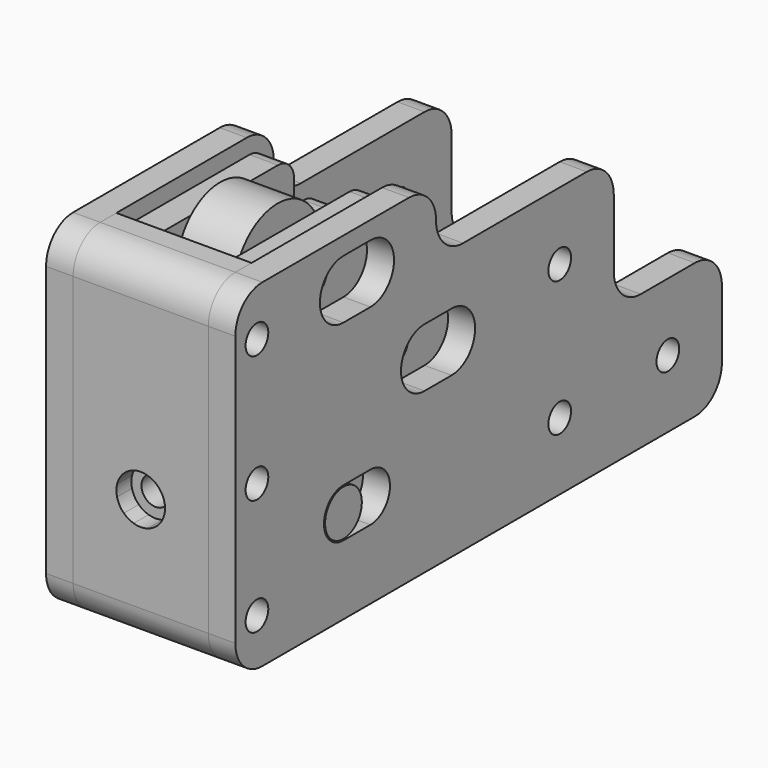
from build123d import *

# Parameters (mm, degrees)
F1_START      = 10
F0_R          = 2.1
F1_DEPTH      = 4
F2_START      = -10
F2_DEPTH      = 4
F3_R          = 8
F3_R_2        = 2.5
F4_DEPTH      = 4.25
F4_DEPTH_BACK = 4.25
F5_DEPTH      = 10
F5_DEPTH_BACK = 10
F6_W          = 3
F6_H          = 39.1219552991
F7_DEPTH      = 9.5
F7_DEPTH_BACK = 9.5
F8_START      = 5.3
F6_R          = 3.4
F6_R_2        = 4.25
F6_R_3        = 2.6
F8_DEPTH      = 4.2
F9_START      = -5.3
F9_DEPTH      = 4.2
F10_START     = 9.5
F10_DEPTH     = 4.5
F11_START     = -9.5
F11_DEPTH     = 4.5
F12_START     = 4.5
F12_DEPTH     = 0.8
F13_START     = -4.5
F13_DEPTH     = 0.8
F14_SIZE      = 0.79999
F15_R         = 2.1
F16_DEPTH     = 56.7675373241
F17_DEPTH     = 47
F18_START     = 54
F18_DEPTH     = 2.7675373241


# Not quite as in the source:
# - a fillet or chamfer is up to 0.001 mm smaller than in the source, because OpenCascade refuses the exact size
# - a feature names something its author has since deleted; it is built from what else it names


with BuildPart() as f1:
    # F0 (on Right) → F1 (new body)
    with BuildSketch(Plane.YZ.offset(F1_START)):
        with BuildLine():
            ThreePointArc((-56.7665373241, -19.1860739807), (-55.30207123, -22.7216078866), (-51.7665373241, -24.1860739807))
            Line((-51.7665373241, -24.1860739807), (-48.7665373241, -24.1860739807))
            Line((-48.7665373241, -24.1860739807), (-48.7665373241, 25.8139260193))
            Line((-48.7665373241, 25.8139260193), (-51.7665373241, 25.8139260193))
            ThreePointArc((-51.7665373241, 25.8139260193), (-55.30207123, 24.3494599252), (-56.7665373241, 20.8139260193))
            Line((-56.7665373241, 20.8139260193), (-56.7665373241, -19.1860739807))
        make_face()
        with Locations((-52.7665373241, -17.1860739807)):
            Circle(F0_R, mode=Mode.SUBTRACT)
        with Locations((-52.7665373241, 0)):
            Circle(F0_R, mode=Mode.SUBTRACT)
        with Locations((-52.7665373241, 18.8139260193)):
            Circle(F0_R, mode=Mode.SUBTRACT)
        with BuildLine():
            Line((-48.7665373241, 25.8139260193), (-48.7665373241, -24.1860739807))
            Line((-48.7665373241, -24.1860739807), (28.2334626759, -24.1860739807))
            ThreePointArc((28.2334626759, -24.1860739807), (31.7689965819, -22.7216078866), (33.2334626759, -19.1860739807))
            Line((33.2334626759, -19.1860739807), (33.2334626759, -9.1860739807))
            ThreePointArc((33.2334626759, -9.1860739807), (31.7689965819, -5.6505400748), (28.2334626759, -4.1860739807))
            Line((28.2334626759, -4.1860739807), (18.2334626759, -4.1860739807))
            ThreePointArc((18.2334626759, -4.1860739807), (14.69792877, -2.7216078866), (13.2334626759, 0.8139260193))
            Line((13.2334626759, 0.8139260193), (13.2334626759, 10.8139260193))
            ThreePointArc((13.2334626759, 10.8139260193), (11.7689965819, 14.3494599252), (8.2334626759, 15.8139260193))
            Line((8.2334626759, 15.8139260193), (-14.6415373241, 15.8139260193))
            ThreePointArc((-14.6415373241, 15.8139260193), (-18.17707123, 17.2783921134), (-19.6415373241, 20.8139260193))
            ThreePointArc((-19.6415373241, 20.8139260193), (-21.1060034181, 24.3494599252), (-24.6415373241, 25.8139260193))
            Line((-24.6415373241, 25.8139260193), (-48.7665373241, 25.8139260193))
        make_face()
        with BuildLine():
            ThreePointArc((-36.7665373241, -13.9080292798), (-40.3665373241, -10.3080292798), (-36.7665373241, -6.7080292798))
            Line((-36.7665373241, -6.7080292798), (-31.7665373241, -6.7080292798))
            ThreePointArc((-31.7665373241, -6.7080292798), (-28.1665373241, -10.3080292798), (-31.7665373241, -13.9080292798))
            Line((-31.7665373241, -13.9080292798), (-36.7665373241, -13.9080292798))
        make_face(mode=Mode.SUBTRACT)
        with Locations((3.2334626759, -14.1860739807)):
            Circle(F0_R, mode=Mode.SUBTRACT)
        with Locations((23.2334626759, -14.1860739807)):
            Circle(F0_R, mode=Mode.SUBTRACT)
        with BuildLine():
            ThreePointArc((-16.7665373241, 8.1639260193), (-12.4165373241, 3.8139260193), (-16.7665373241, -0.5360739807))
            Line((-16.7665373241, -0.5360739807), (-21.7665373241, -0.5360739807))
            ThreePointArc((-21.7665373241, -0.5360739807), (-26.1165373241, 3.8139260193), (-21.7665373241, 8.1639260193))
            Line((-21.7665373241, 8.1639260193), (-16.7665373241, 8.1639260193))
        make_face(mode=Mode.SUBTRACT)
        with BuildLine():
            ThreePointArc((-31.7665373241, 23.1639260193), (-27.4165373241, 18.8139260193), (-31.7665373241, 14.4639260193))
            Line((-31.7665373241, 14.4639260193), (-36.7665373241, 14.4639260193))
            ThreePointArc((-36.7665373241, 14.4639260193), (-41.1165373241, 18.8139260193), (-36.7665373241, 23.1639260193))
            Line((-36.7665373241, 23.1639260193), (-31.7665373241, 23.1639260193))
        make_face(mode=Mode.SUBTRACT)
        with Locations((3.2334626759, 5.8139260193)):
            Circle(F0_R, mode=Mode.SUBTRACT)
    extrude(amount=F1_DEPTH)


with BuildPart() as f2:
    # F0 (on Right) → F2 (new body)
    with BuildSketch(Plane.YZ.offset(F2_START)):
        with BuildLine():
            ThreePointArc((-56.7665373241, -19.1860739807), (-55.30207123, -22.7216078866), (-51.7665373241, -24.1860739807))
            Line((-51.7665373241, -24.1860739807), (-48.7665373241, -24.1860739807))
            Line((-48.7665373241, -24.1860739807), (-48.7665373241, 25.8139260193))
            Line((-48.7665373241, 25.8139260193), (-51.7665373241, 25.8139260193))
            ThreePointArc((-51.7665373241, 25.8139260193), (-55.30207123, 24.3494599252), (-56.7665373241, 20.8139260193))
            Line((-56.7665373241, 20.8139260193), (-56.7665373241, -19.1860739807))
        make_face()
        with Locations((-52.7665373241, -17.1860739807)):
            Circle(F0_R, mode=Mode.SUBTRACT)
        with Locations((-52.7665373241, 0)):
            Circle(F0_R, mode=Mode.SUBTRACT)
        with Locations((-52.7665373241, 18.8139260193)):
            Circle(F0_R, mode=Mode.SUBTRACT)
        with BuildLine():
            Line((-48.7665373241, 25.8139260193), (-48.7665373241, -24.1860739807))
            Line((-48.7665373241, -24.1860739807), (28.2334626759, -24.1860739807))
            ThreePointArc((28.2334626759, -24.1860739807), (31.7689965819, -22.7216078866), (33.2334626759, -19.1860739807))
            Line((33.2334626759, -19.1860739807), (33.2334626759, -9.1860739807))
            ThreePointArc((33.2334626759, -9.1860739807), (31.7689965819, -5.6505400748), (28.2334626759, -4.1860739807))
            Line((28.2334626759, -4.1860739807), (18.2334626759, -4.1860739807))
            ThreePointArc((18.2334626759, -4.1860739807), (14.69792877, -2.7216078866), (13.2334626759, 0.8139260193))
            Line((13.2334626759, 0.8139260193), (13.2334626759, 10.8139260193))
            ThreePointArc((13.2334626759, 10.8139260193), (11.7689965819, 14.3494599252), (8.2334626759, 15.8139260193))
            Line((8.2334626759, 15.8139260193), (-14.6415373241, 15.8139260193))
            ThreePointArc((-14.6415373241, 15.8139260193), (-18.17707123, 17.2783921134), (-19.6415373241, 20.8139260193))
            ThreePointArc((-19.6415373241, 20.8139260193), (-21.1060034181, 24.3494599252), (-24.6415373241, 25.8139260193))
            Line((-24.6415373241, 25.8139260193), (-48.7665373241, 25.8139260193))
        make_face()
        with BuildLine():
            ThreePointArc((-36.7665373241, -13.9080292798), (-40.3665373241, -10.3080292798), (-36.7665373241, -6.7080292798))
            Line((-36.7665373241, -6.7080292798), (-31.7665373241, -6.7080292798))
            ThreePointArc((-31.7665373241, -6.7080292798), (-28.1665373241, -10.3080292798), (-31.7665373241, -13.9080292798))
            Line((-31.7665373241, -13.9080292798), (-36.7665373241, -13.9080292798))
        make_face(mode=Mode.SUBTRACT)
        with Locations((3.2334626759, -14.1860739807)):
            Circle(F0_R, mode=Mode.SUBTRACT)
        with Locations((23.2334626759, -14.1860739807)):
            Circle(F0_R, mode=Mode.SUBTRACT)
        with BuildLine():
            ThreePointArc((-16.7665373241, 8.1639260193), (-12.4165373241, 3.8139260193), (-16.7665373241, -0.5360739807))
            Line((-16.7665373241, -0.5360739807), (-21.7665373241, -0.5360739807))
            ThreePointArc((-21.7665373241, -0.5360739807), (-26.1165373241, 3.8139260193), (-21.7665373241, 8.1639260193))
            Line((-21.7665373241, 8.1639260193), (-16.7665373241, 8.1639260193))
        make_face(mode=Mode.SUBTRACT)
        with BuildLine():
            ThreePointArc((-31.7665373241, 23.1639260193), (-27.4165373241, 18.8139260193), (-31.7665373241, 14.4639260193))
            Line((-31.7665373241, 14.4639260193), (-36.7665373241, 14.4639260193))
            ThreePointArc((-36.7665373241, 14.4639260193), (-41.1165373241, 18.8139260193), (-36.7665373241, 23.1639260193))
            Line((-36.7665373241, 23.1639260193), (-31.7665373241, 23.1639260193))
        make_face(mode=Mode.SUBTRACT)
        with Locations((3.2334626759, 5.8139260193)):
            Circle(F0_R, mode=Mode.SUBTRACT)
    extrude(amount=-F2_DEPTH)


with BuildPart() as f4:
    # F3 (on Right) → F4 (new body, two sides)
    with BuildSketch(Plane.YZ) as f4_sk:
        with Locations((-36.7665373241, 18.8139260193)):
            Circle(F3_R)
        with Locations((-36.7665373241, 18.8139260193)):
            Circle(F3_R_2, mode=Mode.SUBTRACT)
    extrude(amount=F4_DEPTH)
    extrude(f4_sk.sketch, amount=-F4_DEPTH_BACK)


with BuildPart() as f4b:
    # F3 (on Right) → F4, piece 2 (new body, two sides)
    with BuildSketch(Plane.YZ) as f4_2_sk:
        with Locations((-21.7665373241, 3.8139260193)):
            Circle(F3_R)
        with Locations((-21.7665373241, 3.8139260193)):
            Circle(F3_R_2, mode=Mode.SUBTRACT)
    extrude(amount=F4_DEPTH)
    extrude(f4_2_sk.sketch, amount=-F4_DEPTH_BACK)


with BuildPart() as f5:
    # F0 (on Right) → F5 (new body, two sides)
    with BuildSketch(Plane.YZ) as f5_sk:
        with BuildLine():
            ThreePointArc((-56.7665373241, -19.1860739807), (-55.30207123, -22.7216078866), (-51.7665373241, -24.1860739807))
            Line((-51.7665373241, -24.1860739807), (-48.7665373241, -24.1860739807))
            Line((-48.7665373241, -24.1860739807), (-48.7665373241, 25.8139260193))
            Line((-48.7665373241, 25.8139260193), (-51.7665373241, 25.8139260193))
            ThreePointArc((-51.7665373241, 25.8139260193), (-55.30207123, 24.3494599252), (-56.7665373241, 20.8139260193))
            Line((-56.7665373241, 20.8139260193), (-56.7665373241, -19.1860739807))
        make_face()
        with Locations((-52.7665373241, -17.1860739807)):
            Circle(F0_R, mode=Mode.SUBTRACT)
        with Locations((-52.7665373241, 0)):
            Circle(F0_R, mode=Mode.SUBTRACT)
        with Locations((-52.7665373241, 18.8139260193)):
            Circle(F0_R, mode=Mode.SUBTRACT)
    extrude(amount=-F5_DEPTH)
    extrude(f5_sk.sketch, amount=F5_DEPTH_BACK)


with BuildPart() as f7:
    # F6 (on Right) → F7 (new body, two sides)
    with BuildSketch(Plane.YZ) as f7_sk:
        with Locations((-47.2665373241, 4.2529483698)):
            Rectangle(F6_W, F6_H)
    extrude(amount=F7_DEPTH)
    extrude(f7_sk.sketch, amount=-F7_DEPTH_BACK)

    # F6 (on Right) → F8 (join)
    with BuildSketch(Plane.YZ.offset(F8_START)):
        with BuildLine():
            Line((-45.7665373241, 23.8139260193), (-45.7665373241, -15.3080292798))
            Line((-45.7665373241, -15.3080292798), (-16.7278158617, -15.3080292798))
            ThreePointArc((-16.7278158617, -15.3080292798), (-13.4191378014, -14.0567156487), (-11.7665373241, -10.9290890769))
            Line((-11.7665373241, -10.9290890769), (-11.7665373241, 10.8139260193))
            ThreePointArc((-11.7665373241, 10.8139260193), (-12.6452169805, 12.9352463629), (-14.7665373241, 13.8139260193))
            Line((-14.7665373241, 13.8139260193), (-18.7665373241, 13.8139260193))
            ThreePointArc((-18.7665373241, 13.8139260193), (-20.8878576676, 14.6926056757), (-21.7665373241, 16.8139260193))
            Line((-21.7665373241, 16.8139260193), (-21.7665373241, 20.8139260193))
            ThreePointArc((-21.7665373241, 20.8139260193), (-22.6452169805, 22.9352463629), (-24.7665373241, 23.8139260193))
            Line((-24.7665373241, 23.8139260193), (-45.7665373241, 23.8139260193))
        make_face()
        with Locations((-36.7665373241, -10.3080292798)):
            Circle(F6_R, mode=Mode.SUBTRACT)
        with Locations((-21.7665373241, 3.8139260193)):
            Circle(F6_R_2, mode=Mode.SUBTRACT)
        with Locations((-36.7665373241, 18.8139260193)):
            Circle(F6_R_2, mode=Mode.SUBTRACT)
        with Locations((-36.7665373241, 18.8139260193)):
            Circle(F6_R_2)
        with Locations((-36.7665373241, 18.8139260193)):
            Circle(F6_R_3, mode=Mode.SUBTRACT)
        with Locations((-21.7665373241, 3.8139260193)):
            Circle(F6_R_2)
        with Locations((-21.7665373241, 3.8139260193)):
            Circle(F6_R_3, mode=Mode.SUBTRACT)
        with Locations((-36.7665373241, -10.3080292798)):
            Circle(F6_R)
    extrude(amount=F8_DEPTH)

    # F6 (on Right) → F9 (join)
    with BuildSketch(Plane.YZ.offset(F9_START)):
        with BuildLine():
            Line((-45.7665373241, 23.8139260193), (-45.7665373241, -15.3080292798))
            Line((-45.7665373241, -15.3080292798), (-16.7278158617, -15.3080292798))
            ThreePointArc((-16.7278158617, -15.3080292798), (-13.4191378014, -14.0567156487), (-11.7665373241, -10.9290890769))
            Line((-11.7665373241, -10.9290890769), (-11.7665373241, 10.8139260193))
            ThreePointArc((-11.7665373241, 10.8139260193), (-12.6452169805, 12.9352463629), (-14.7665373241, 13.8139260193))
            Line((-14.7665373241, 13.8139260193), (-18.7665373241, 13.8139260193))
            ThreePointArc((-18.7665373241, 13.8139260193), (-20.8878576676, 14.6926056757), (-21.7665373241, 16.8139260193))
            Line((-21.7665373241, 16.8139260193), (-21.7665373241, 20.8139260193))
            ThreePointArc((-21.7665373241, 20.8139260193), (-22.6452169805, 22.9352463629), (-24.7665373241, 23.8139260193))
            Line((-24.7665373241, 23.8139260193), (-45.7665373241, 23.8139260193))
        make_face()
        with Locations((-36.7665373241, -10.3080292798)):
            Circle(F6_R, mode=Mode.SUBTRACT)
        with Locations((-21.7665373241, 3.8139260193)):
            Circle(F6_R_2, mode=Mode.SUBTRACT)
        with Locations((-36.7665373241, 18.8139260193)):
            Circle(F6_R_2, mode=Mode.SUBTRACT)
        with Locations((-36.7665373241, 18.8139260193)):
            Circle(F6_R_2)
        with Locations((-36.7665373241, 18.8139260193)):
            Circle(F6_R_3, mode=Mode.SUBTRACT)
        with Locations((-21.7665373241, 3.8139260193)):
            Circle(F6_R_2)
        with Locations((-21.7665373241, 3.8139260193)):
            Circle(F6_R_3, mode=Mode.SUBTRACT)
        with Locations((-36.7665373241, -10.3080292798)):
            Circle(F6_R)
    extrude(amount=-F9_DEPTH)

    # F6 (on Right) → F10 (join)
    with BuildSketch(Plane.YZ.offset(F10_START)):
        with Locations((-36.7665373241, -10.3080292798)):
            Circle(F6_R)
    extrude(amount=F10_DEPTH)

    # F6 (on Right) → F11 (join)
    with BuildSketch(Plane.YZ.offset(F11_START)):
        with Locations((-36.7665373241, -10.3080292798)):
            Circle(F6_R)
    extrude(amount=-F11_DEPTH)

    # F6 (on Right) → F12 (join)
    with BuildSketch(Plane.YZ.offset(F12_START)):
        with Locations((-36.7665373241, 18.8139260193)):
            Circle(F6_R_2)
        with Locations((-36.7665373241, 18.8139260193)):
            Circle(F6_R_3, mode=Mode.SUBTRACT)
        with Locations((-21.7665373241, 3.8139260193)):
            Circle(F6_R_2)
        with Locations((-21.7665373241, 3.8139260193)):
            Circle(F6_R_3, mode=Mode.SUBTRACT)
    extrude(amount=F12_DEPTH)

    # F6 (on Right) → F13 (join)
    with BuildSketch(Plane.YZ.offset(F13_START)):
        with Locations((-36.7665373241, 18.8139260193)):
            Circle(F6_R_2)
        with Locations((-36.7665373241, 18.8139260193)):
            Circle(F6_R_3, mode=Mode.SUBTRACT)
        with Locations((-21.7665373241, 3.8139260193)):
            Circle(F6_R_2)
        with Locations((-21.7665373241, 3.8139260193)):
            Circle(F6_R_3, mode=Mode.SUBTRACT)
    extrude(amount=-F13_DEPTH)

    # F14 (size 0.8 in the source; OpenCascade refuses exactly that, so slightly less here)
    f14_edges = [f7.edges().sort_by_distance(p)[0] for p in [
        (-4.5, -41.016537, 18.813926),
        (-4.5, -26.016537, 3.813926),
        (4.5, -26.016537, 3.813926),
        (4.5, -41.016537, 18.813926),
    ]]
    chamfer(f14_edges, length=F14_SIZE)


with BuildPart() as f16_tool:
    # F15 (on Front) → F16 (new body, through all)
    with BuildSketch(Plane.XZ):
        with Locations((0, -5)):
            Circle(F15_R)
    extrude(amount=F16_DEPTH)


with BuildPart() as f5_1:
    add(f5.part)

    # F16: cut by f16_tool
    add(f16_tool.part, mode=Mode.SUBTRACT)

    # F15 (on Front) → F18 (cut)
    with BuildSketch(Plane.XZ.offset(F18_START)):
        with BuildLine():
            Line((3.4940315146, -5.8670315881), (3.5057978621, -4.1818427105))
            ThreePointArc((3.5057978621, -4.1818427105), (3.1301831374, -3.2218117293), (2.4978871385, -2.4075957407))
            Line((2.4978871385, -2.4075957407), (1.044353934, -1.5548113462))
            ThreePointArc((1.044353934, -1.5548113462), (0.0251353535, -1.4000877491), (-0.9961443762, -1.5405641527))
            Line((-0.9961443762, -1.5405641527), (-2.461443928, -2.3729686357))
            ThreePointArc((-2.461443928, -2.3729686357), (-3.1050477839, -3.1782760199), (-3.4940315146, -4.1329684119))
            Line((-3.4940315146, -4.1329684119), (-3.5057978621, -5.8181572895))
            ThreePointArc((-3.5057978621, -5.8181572895), (-3.1301831374, -6.7781882707), (-2.4978871385, -7.5924042593))
            Line((-2.4978871385, -7.5924042593), (-1.044353934, -8.4451886538))
            ThreePointArc((-1.044353934, -8.4451886538), (-0.0251353535, -8.5999122509), (0.9961443762, -8.4594358473))
            Line((0.9961443762, -8.4594358473), (2.461443928, -7.6270313643))
            ThreePointArc((2.461443928, -7.6270313643), (3.1050477839, -6.8217239801), (3.4940315146, -5.8670315881))
        make_face()
        with Locations((0, -5)):
            Circle(F15_R, mode=Mode.SUBTRACT)
        with BuildLine():
            Line((-3.5057978621, -5.8181572895), (-3.4940315146, -4.1329684119))
            ThreePointArc((-3.4940315146, -4.1329684119), (-3.5999122509, -4.9748646465), (-3.5057978621, -5.8181572895))
        make_face()
        with BuildLine():
            Line((-2.461443928, -2.3729686357), (-0.9961443762, -1.5405641527))
            ThreePointArc((-0.9961443762, -1.5405641527), (-1.7781882707, -1.8698168626), (-2.461443928, -2.3729686357))
        make_face()
        with BuildLine():
            Line((1.044353934, -1.5548113462), (2.4978871385, -2.4075957407))
            ThreePointArc((2.4978871385, -2.4075957407), (1.8217239801, -1.8949522161), (1.044353934, -1.5548113462))
        make_face()
        with BuildLine():
            ThreePointArc((3.4940315146, -5.8670315881), (3.5734096779, -5.4367416555), (3.6, -5))
            ThreePointArc((3.6, -5), (3.5763719258, -4.5882186888), (3.5057978621, -4.1818427105))
            Line((3.5057978621, -4.1818427105), (3.4940315146, -5.8670315881))
        make_face()
        with BuildLine():
            ThreePointArc((0.9961443762, -8.4594358473), (1.7781882707, -8.1301831374), (2.461443928, -7.6270313643))
            Line((2.461443928, -7.6270313643), (0.9961443762, -8.4594358473))
        make_face()
        with BuildLine():
            ThreePointArc((-2.4978871385, -7.5924042593), (-1.8217239801, -8.1050477839), (-1.044353934, -8.4451886538))
            Line((-1.044353934, -8.4451886538), (-2.4978871385, -7.5924042593))
        make_face()
    extrude(amount=F18_DEPTH, mode=Mode.SUBTRACT)


with BuildPart() as f7_1:
    add(f7.part)

    # F16: cut by f16_tool
    add(f16_tool.part, mode=Mode.SUBTRACT)

    # F15 (on Front) → F17 (cut)
    with BuildSketch(Plane.XZ):
        with BuildLine():
            ThreePointArc((-3.4940315146, -4.1329684119), (-3.1050477839, -3.1782760199), (-2.461443928, -2.3729686357))
            Line((-2.461443928, -2.3729686357), (-3.4858058936, -2.9548861633))
            Line((-3.4858058936, -2.9548861633), (-3.4940315146, -4.1329684119))
        make_face()
        with BuildLine():
            ThreePointArc((-0.9961443762, -1.5405641527), (0.0251353535, -1.4000877491), (1.044353934, -1.5548113462))
            Line((1.044353934, -1.5548113462), (0.0282175894, -0.9586466251))
            Line((0.0282175894, -0.9586466251), (-0.9961443762, -1.5405641527))
        make_face()
        with BuildLine():
            ThreePointArc((2.4978871385, -2.4075957407), (3.1301831374, -3.2218117293), (3.5057978621, -4.1818427105))
            Line((3.5057978621, -4.1818427105), (3.5140234831, -3.0037604618))
            Line((3.5140234831, -3.0037604618), (2.4978871385, -2.4075957407))
        make_face()
        with BuildLine():
            Line((3.4858058936, -7.0451138367), (3.4940315146, -5.8670315881))
            ThreePointArc((3.4940315146, -5.8670315881), (3.1050477839, -6.8217239801), (2.461443928, -7.6270313643))
            Line((2.461443928, -7.6270313643), (3.4858058936, -7.0451138367))
        make_face()
        with BuildLine():
            Line((-3.5140234831, -6.9962395382), (-2.4978871385, -7.5924042593))
            ThreePointArc((-2.4978871385, -7.5924042593), (-3.1301831374, -6.7781882707), (-3.5057978621, -5.8181572895))
            Line((-3.5057978621, -5.8181572895), (-3.5140234831, -6.9962395382))
        make_face()
        with BuildLine():
            Line((-0.0282175894, -9.0413533749), (0.9961443762, -8.4594358473))
            ThreePointArc((0.9961443762, -8.4594358473), (-0.0251353535, -8.5999122509), (-1.044353934, -8.4451886538))
            Line((-1.044353934, -8.4451886538), (-0.0282175894, -9.0413533749))
        make_face()
        with BuildLine():
            Line((3.4940315146, -5.8670315881), (3.5057978621, -4.1818427105))
            ThreePointArc((3.5057978621, -4.1818427105), (3.1301831374, -3.2218117293), (2.4978871385, -2.4075957407))
            Line((2.4978871385, -2.4075957407), (1.044353934, -1.5548113462))
            ThreePointArc((1.044353934, -1.5548113462), (0.0251353535, -1.4000877491), (-0.9961443762, -1.5405641527))
            Line((-0.9961443762, -1.5405641527), (-2.461443928, -2.3729686357))
            ThreePointArc((-2.461443928, -2.3729686357), (-3.1050477839, -3.1782760199), (-3.4940315146, -4.1329684119))
            Line((-3.4940315146, -4.1329684119), (-3.5057978621, -5.8181572895))
            ThreePointArc((-3.5057978621, -5.8181572895), (-3.1301831374, -6.7781882707), (-2.4978871385, -7.5924042593))
            Line((-2.4978871385, -7.5924042593), (-1.044353934, -8.4451886538))
            ThreePointArc((-1.044353934, -8.4451886538), (-0.0251353535, -8.5999122509), (0.9961443762, -8.4594358473))
            Line((0.9961443762, -8.4594358473), (2.461443928, -7.6270313643))
            ThreePointArc((2.461443928, -7.6270313643), (3.1050477839, -6.8217239801), (3.4940315146, -5.8670315881))
        make_face()
        with Locations((0, -5)):
            Circle(F15_R, mode=Mode.SUBTRACT)
        with Locations((0, -5)):
            Circle(F15_R)
    extrude(amount=F17_DEPTH, mode=Mode.SUBTRACT)


solid = Compound([f1.part, f2.part, f4.part, f4b.part, f5_1.part, f7_1.part])
